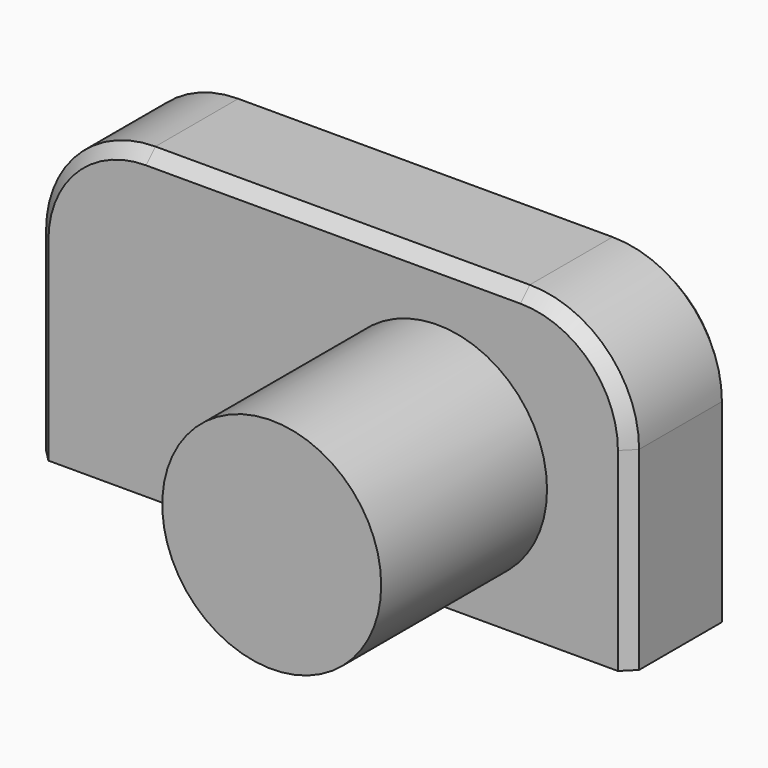
from build123d import *

# Parameters (mm, degrees)
F0_W         = 256.1325952411
F0_H         = 131.0712322593
F1_DEPTH     = 54.864
F2_R         = 47.2171888529
F3_SIZE      = 5.08
F4_SIZE      = 5.08
F5_R         = 47.2807680991
F6_DEPTH     = 25.4
F7_TEXT_SIZE = 35.2240911764
F8_DEPTH     = 1.016
F9_DEPTH     = 24.13
F10_DEPTH    = 40


# Not quite as in the source:
# - Text() gives the source's letters only with a copy of the font that has no kerning and outlines rounded to 1/6400 em; it was checked with that copy


with BuildPart() as f1:
    # F0 (on Front) → F1 (new body)
    with BuildSketch(Plane.XZ):
        with Locations((34.1411419213, 5.4177083075)):
            Rectangle(F0_W, F0_H)
    extrude(amount=F1_DEPTH)

    # F2
    f2_edges = [f1.edges().sort_by_distance(p)[0] for p in [
        (162.20744, -27.432, 70.953324),
        (-93.925156, -27.432, 70.953324),
    ]]
    fillet(f2_edges, radius=F2_R)

    # F3
    f3_edges = [f1.edges().sort_by_distance(p)[0] for p in [
        (148.377845, -54.864, 57.12373),
    ]]
    chamfer(f3_edges, length=F3_SIZE)

    # F4
    f4_edges = [f1.edges().sort_by_distance(p)[0] for p in [
        (34.141142, 0, 70.953324),
        (148.377845, 0, 57.12373),
        (-80.095561, 0, 57.12373),
        (162.20744, 0, -18.190886),
        (-93.925156, 0, -18.190886),
        (34.141142, 0, -60.117908),
    ]]
    chamfer(f4_edges, length=F4_SIZE)

    # F5 (on face) → F6 (join)
    with BuildSketch(Plane.XZ.offset(54.864)):
        with Locations((79.2201682925, -1.0698497063)):
            Circle(F5_R)
    extrude(amount=F6_DEPTH)

    # F7 (on face) → F8 (join)
    with BuildSketch(Plane(origin=(0, 0, 0), x_dir=(-1, 0, 0), z_dir=(0, 1, 0))):
        with Locations((-157.1274395418, -55.0379078221)):
            Text('NIKE', F7_TEXT_SIZE, font='Open Sans', text_align=(TextAlign.LEFT, TextAlign.BOTTOM))
    extrude(amount=F8_DEPTH)

    # F9 (add): a face of the model
    f9_faces = [f1.faces().sort_by_distance(p)[0] for p in [
        (79.2201682925, -80.264, -1.0698497063),
    ]]
    extrude(f9_faces, amount=F9_DEPTH)

    # F10 (add): a face of the model
    f10_faces = [f1.faces().sort_by_distance(p)[0] for p in [
        (79.2201682925, -104.394, -1.0698497063),
    ]]
    extrude(f10_faces, amount=F10_DEPTH)


solid = f1.part
